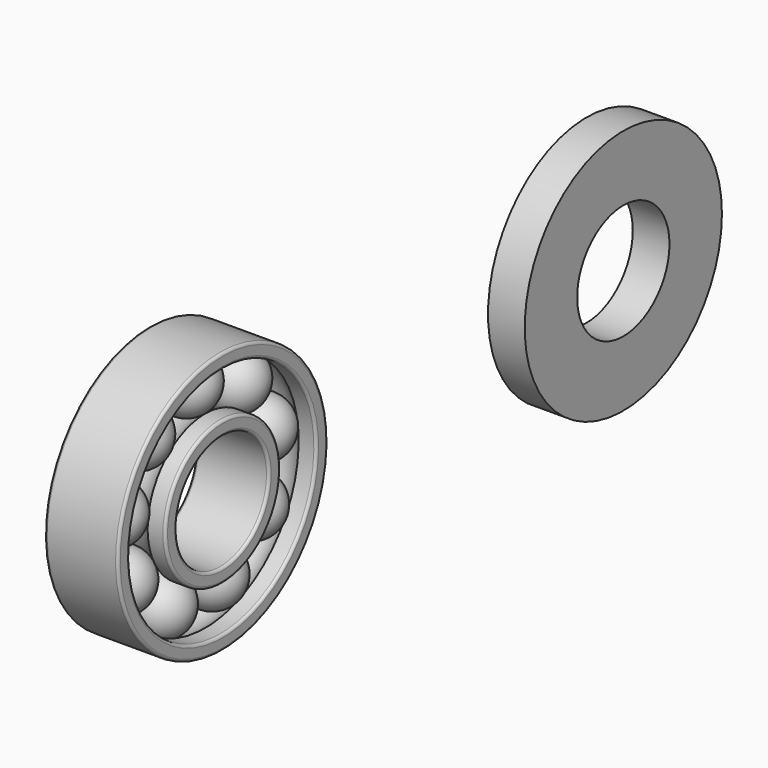
from build123d import *

# Parameters (mm, degrees)
F9_COUNT = 9


with BuildPart() as f6:
    # F5 (on Front) → F6 (revolve)
    with BuildSketch(Plane.XZ):
        with BuildLine():
            ThreePointArc((-7, 11.5), (-6.8535533906, 11.1464466094), (-6.5, 11))
            Line((-6.5, 11), (6.5, 11))
            ThreePointArc((6.5, 11), (6.8535533906, 11.1464466094), (7, 11.5))
            Line((7, 11.5), (7, 13.2109358311))
            ThreePointArc((7, 13.2109358311), (6.8535533906, 13.5644892217), (6.5, 13.7109358311))
            Line((6.5, 13.7109358311), (3.6005455913, 13.7109358311))
            ThreePointArc((3.6005455913, 13.7109358311), (0, 12.4), (-3.6005455913, 13.7109358311))
            Line((-3.6005455913, 13.7109358311), (-6.5, 13.7109358311))
            ThreePointArc((-6.5, 13.7109358311), (-6.8535533906, 13.5644892217), (-7, 13.2109358311))
            Line((-7, 13.2109358311), (-7, 11.5))
        make_face()
    revolve(axis=Axis((0.2612321927, 0, 0), (1, 0, 0)))


with BuildPart() as f6b:
    # F5 (on Front) → F6, piece 2 (revolve)
    with BuildSketch(Plane.XZ):
        with BuildLine():
            Line((-6.5, 22.2890641689), (-3.6005455913, 22.2890641689))
            ThreePointArc((-3.6005455913, 22.2890641689), (0, 23.6), (3.6005455913, 22.2890641689))
            Line((3.6005455913, 22.2890641689), (6.5, 22.2890641689))
            ThreePointArc((6.5, 22.2890641689), (6.8535533906, 22.4355107783), (7, 22.7890641689))
            Line((7, 22.7890641689), (7, 24.5))
            ThreePointArc((7, 24.5), (6.8535533906, 24.8535533906), (6.5, 25))
            Line((6.5, 25), (-6.5, 25))
            ThreePointArc((-6.5, 25), (-6.8535533906, 24.8535533906), (-7, 24.5))
            Line((-7, 24.5), (-7, 22.7890641689))
            ThreePointArc((-7, 22.7890641689), (-6.8535533906, 22.4355107783), (-6.5, 22.2890641689))
        make_face()
    revolve(axis=Axis((0.2612321927, 0, 0), (1, 0, 0)))


with BuildPart() as f8:
    # F7 (on Front) → F8 (revolve)
    with BuildSketch(Plane.XZ):
        with BuildLine():
            ThreePointArc((5.6, 18), (0, 23.6), (-5.6, 18))
            Line((-5.6, 18), (5.6, 18))
        make_face()
    revolve(axis=Axis((0.4027837024, 0, 18), (1, 0, 0)))


with BuildPart() as f9_1:
    # F9: instance of F8
    add(f8.part.rotate(Axis((6.5, 0, 0), (1, 0, 0)), 1 * 360 / F9_COUNT))


with BuildPart() as f9_2:
    # F9: instance of F8
    add(f8.part.rotate(Axis((6.5, 0, 0), (1, 0, 0)), 2 * 360 / F9_COUNT))


with BuildPart() as f9_3:
    # F9: instance of F8
    add(f8.part.rotate(Axis((6.5, 0, 0), (1, 0, 0)), 3 * 360 / F9_COUNT))


with BuildPart() as f9_4:
    # F9: instance of F8
    add(f8.part.rotate(Axis((6.5, 0, 0), (1, 0, 0)), 4 * 360 / F9_COUNT))


with BuildPart() as f9_5:
    # F9: instance of F8
    add(f8.part.rotate(Axis((6.5, 0, 0), (1, 0, 0)), 5 * 360 / F9_COUNT))


with BuildPart() as f9_6:
    # F9: instance of F8
    add(f8.part.rotate(Axis((6.5, 0, 0), (1, 0, 0)), 6 * 360 / F9_COUNT))


with BuildPart() as f9_7:
    # F9: instance of F8
    add(f8.part.rotate(Axis((6.5, 0, 0), (1, 0, 0)), 7 * 360 / F9_COUNT))


with BuildPart() as f9_8:
    # F9: instance of F8
    add(f8.part.rotate(Axis((6.5, 0, 0), (1, 0, 0)), 8 * 360 / F9_COUNT))


with BuildPart() as f11:
    # F10 (on Top) → F11 (revolve)
    with BuildSketch(Plane.XY):
        Polygon((0, 108.9236316694), (0, 106.4236316694), (7, 106.4236316694), (7, 118.9236316694), (0, 118.9236316694), (0, 115.1736316694), (4.6666666667, 115.1736316694), (4.6666666667, 108.9236316694), align=None)
    revolve(axis=Axis((1.000135277, 95.4236316694, 0), (1, 0, 0)))


solid = Compound([f6.part, f6b.part, f8.part, f9_1.part, f9_2.part, f9_3.part, f9_4.part, f9_5.part, f9_6.part, f9_7.part, f9_8.part, f11.part])
